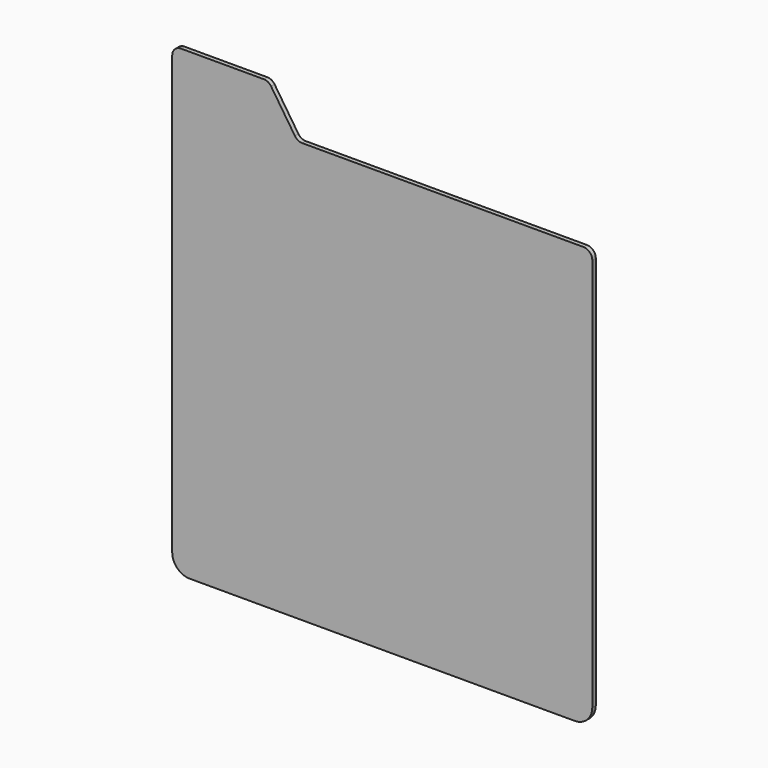
from build123d import *

# Parameters (mm, degrees)
F1_DEPTH = 1.5875
F2_R     = 6.35
F3_R     = 12.7


with BuildPart() as f1:
    # F0 (on Front) → F1 (new body, symmetric)
    with BuildSketch(Plane.XZ):
        Polygon((-152.4, 152.4), (-152.4, -152.4), (152.4, -152.4), (152.4, 152.4), (-61.4666454494, 152.4), (-82.55, 184.15), (-152.4, 184.15), align=None)
    extrude(amount=F1_DEPTH, both=True)

    # F2
    f2_edges = [f1.edges().sort_by_distance(p)[0] for p in [
        (152.4, 0, 152.4),
        (-152.4, 0, 184.15),
        (-61.466645, 0, 152.4),
        (-82.55, 0, 184.15),
    ]]
    fillet(f2_edges, radius=F2_R)

    # F3
    f3_edges = [f1.edges().sort_by_distance(p)[0] for p in [
        (152.4, 0, -152.4),
        (-152.4, 0, -152.4),
    ]]
    fillet(f3_edges, radius=F3_R)


solid = f1.part
